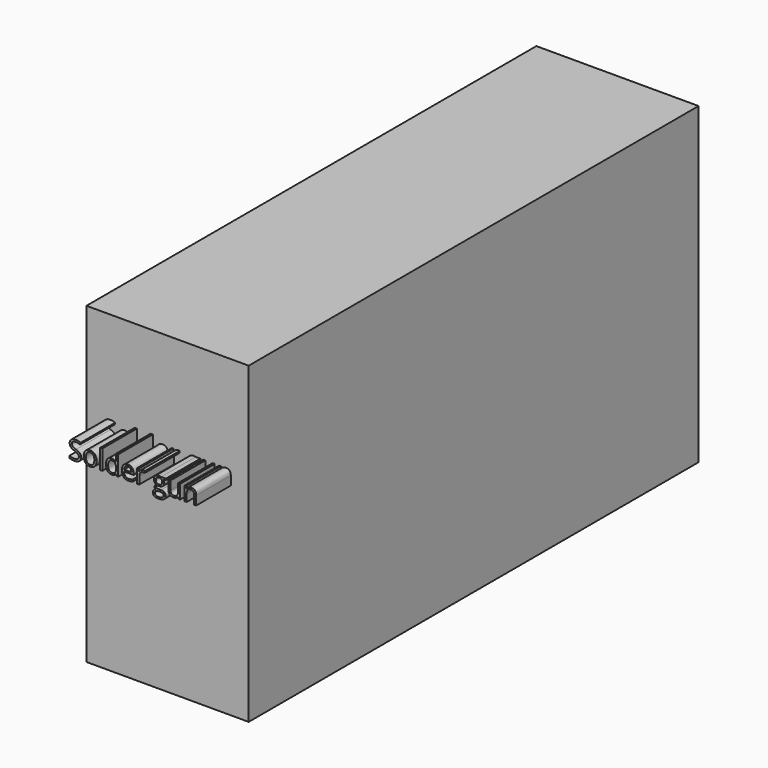
from build123d import *

# Parameters (mm, degrees)
F0_W         = 95.25
F0_H         = 184.15
F1_DEPTH     = 330.2
F2_TEXT_SIZE = 15.216699429
F3_DEPTH     = 25.4


# Not quite as in the source:
# - Text() gives the source's letters only with a copy of the font that has no kerning and outlines rounded to 1/6400 em; it was checked with that copy


with BuildPart() as f1:
    # F0 (on Front) → F1 (new body)
    with BuildSketch(Plane.XZ):
        Rectangle(F0_W, F0_H)
    extrude(amount=F1_DEPTH)

    # F2 (on face) → F3 (join)
    with BuildSketch(Plane.XZ.offset(330.2)):
        with Locations((-38.1, 26.6736234484)):
            Text('Solder gun', F2_TEXT_SIZE, font='Open Sans', text_align=(TextAlign.LEFT, TextAlign.BOTTOM))
    extrude(amount=F3_DEPTH)


solid = f1.part
